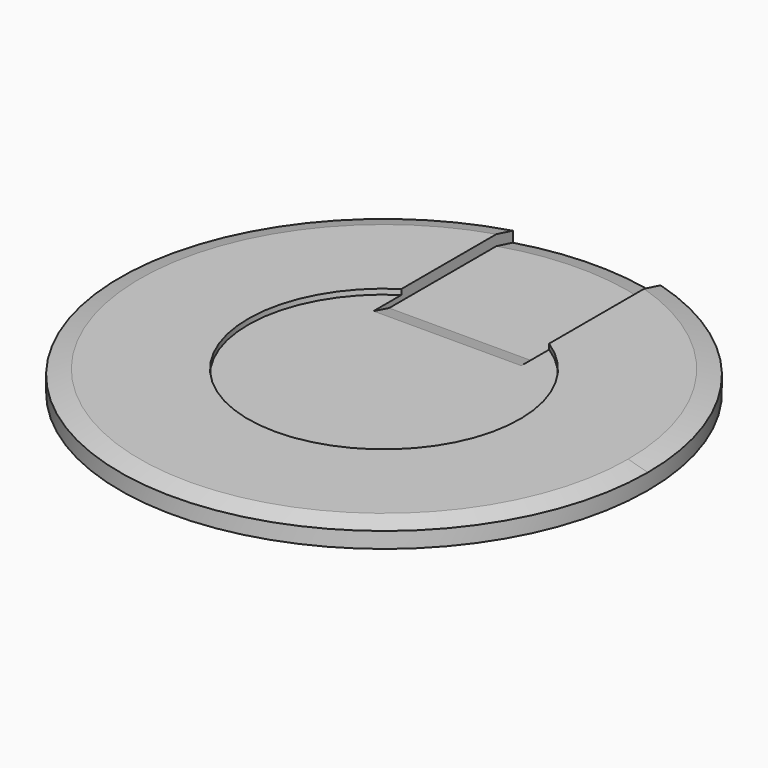
from build123d import *

# Parameters (mm, degrees)
F0_R     = 50
F1_DEPTH = 4
F2_R     = 25.75
F3_DEPTH = 1
F5_DEPTH = 2
F6_SIZE2 = 3.732041
F6_SIZE  = 0.99999


# Not quite as in the source:
# - a fillet or chamfer is up to 0.001 mm smaller than in the source, because OpenCascade refuses the exact size
# - a feature names something its author has since deleted; it is built from what else it names


with BuildPart() as f1:
    # F0 (on Top) → F1 (new body)
    with BuildSketch(Plane.XY):
        Circle(F0_R)
    extrude(amount=F1_DEPTH)

    # F2 (on face) → F3 (cut)
    with BuildSketch(Plane.XY.offset(4)):
        Circle(F2_R)
    extrude(amount=-F3_DEPTH, mode=Mode.SUBTRACT)

    # F4 (on face) → F5 (cut)
    with BuildSketch(Plane.XY.offset(4)):
        with BuildLine():
            Line((-14, 21.6116288141), (-14, 15))
            Line((-14, 15), (14, 15))
            Line((14, 15), (14, 21.6116288141))
            ThreePointArc((14, 21.6116288141), (0, 25.75), (-14, 21.6116288141))
        make_face()
        with BuildLine():
            Line((-14, 48), (-14, 21.6116288141))
            ThreePointArc((-14, 21.6116288141), (0, 25.75), (14, 21.6116288141))
            Line((14, 21.6116288141), (14, 48))
            ThreePointArc((14, 48), (0, 50), (-14, 48))
        make_face()
        with BuildLine():
            Line((-14, 55), (-14, 48))
            ThreePointArc((-14, 48), (0, 50), (14, 48))
            Line((14, 48), (14, 55))
            Line((14, 55), (-14, 55))
        make_face()
    extrude(amount=-F5_DEPTH, mode=Mode.SUBTRACT)

    # F6 (size 1 and 3.7320508076 in the source; OpenCascade refuses exactly that, so slightly less here)
    f6_edges = [f1.edges().sort_by_distance(p)[0] for p in [
        (0, 15, 2),
        (-30, -40, 4),
        (0, 50, 2),
        (40, 30, 4),
    ]]
    chamfer(f6_edges, length=F6_SIZE, length2=F6_SIZE2)


solid = f1.part
